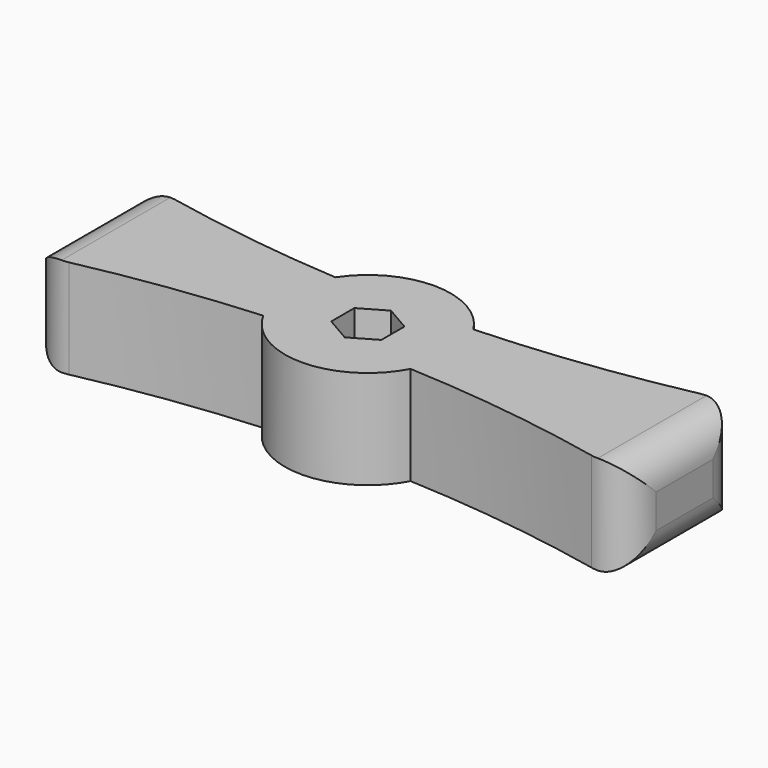
from build123d import *

# Parameters (mm, degrees)
F1_DEPTH = 15.494
F2_R     = 5.08
F4_DEPTH = 15.495


# Not quite as in the source:
# - a feature names something its author has since deleted; it is built from what else it names


with BuildPart() as f1:
    # F0 (on Top) → F1 (new body)
    with BuildSketch(Plane.XY):
        with BuildLine():
            ThreePointArc((-10.8447933041, 7.1841250258), (-28.0007995808, 9.0295397064), (-44.9371226132, 12.3303076252))
            Line((-44.9371226132, 12.3303076252), (-44.9371226132, -11.5082878619))
            ThreePointArc((-44.9371226132, -11.5082878619), (-28.2764136106, -8.174493828), (-11.391166434, -6.2819202055))
            ThreePointArc((-11.391166434, -6.2819202055), (-12.9978101968, 0.5273748986), (-10.8447933041, 7.1841250258))
        make_face()
        with BuildLine():
            ThreePointArc((10.9930542238, 6.9551386059), (0.1363965549, 13.007789596), (-10.8447933041, 7.1841250258))
            ThreePointArc((-10.8447933041, 7.1841250258), (0.0710380129, 6.7747130853), (10.9930542238, 6.9551386059))
        make_face()
        with BuildLine():
            ThreePointArc((10.9930542238, 6.9551386059), (0.0710380129, 6.7747130853), (-10.8447933041, 7.1841250258))
            ThreePointArc((-10.8447933041, 7.1841250258), (-12.9978101968, 0.5273748986), (-11.391166434, -6.2819202055))
            ThreePointArc((-11.391166434, -6.2819202055), (0.0626903929, -5.8267272063), (11.5236895742, -6.035376773))
            ThreePointArc((11.5236895742, -6.035376773), (12.6318479257, -3.1076698953), (13.0085046871, 0))
            ThreePointArc((13.0085046871, 0), (12.4944866159, 3.6206350823), (10.9930542238, 6.9551386059))
        make_face()
        with BuildLine():
            ThreePointArc((11.5236895742, -6.035376773), (0.0626903929, -5.8267272063), (-11.391166434, -6.2819202055))
            ThreePointArc((-11.391166434, -6.2819202055), (0.1399518192, -13.0077518305), (11.5236895742, -6.035376773))
        make_face()
        with BuildLine():
            ThreePointArc((49.3212305009, 12.3303076252), (30.2859906696, 8.7239574701), (10.9930542238, 6.9551386059))
            ThreePointArc((10.9930542238, 6.9551386059), (12.4944866159, 3.6206350823), (13.0085046871, 0))
            ThreePointArc((13.0085046871, 0), (12.6318479257, -3.1076698953), (11.5236895742, -6.035376773))
            ThreePointArc((11.5236895742, -6.035376773), (30.5547762597, -7.8580173956), (49.3212305009, -11.5082878619))
            Line((49.3212305009, -11.5082878619), (49.3212305009, 12.3303076252))
        make_face()
    extrude(amount=F1_DEPTH)

    # F2
    f2_edges = [f1.edges().sort_by_distance(p)[0] for p in [
        (-44.937123, 0.41101, 15.494),
        (49.321231, 0.41101, 15.494),
        (-44.937123, 0.41101, 0),
        (49.321231, 0.41101, 0),
        (-44.937123, 12.330308, 7.747),
        (-44.937123, -11.508288, 7.747),
        (49.321231, -11.508288, 7.747),
        (49.321231, 12.330308, 7.747),
    ]]
    fillet(f2_edges, radius=F2_R)

    # F3 (on face) → F4 (cut, through all)
    with BuildSketch(Plane.XY.offset(15.494)):
        Polygon((3.9274184965, -2.2674961262), (3.9274184965, 2.2674961262), (0, 4.5349922523), (-3.9274184965, 2.2674961262), (-3.9274184965, -2.2674961262), (0, -4.5349922523), align=None)
    extrude(amount=-F4_DEPTH, mode=Mode.SUBTRACT)


solid = f1.part
